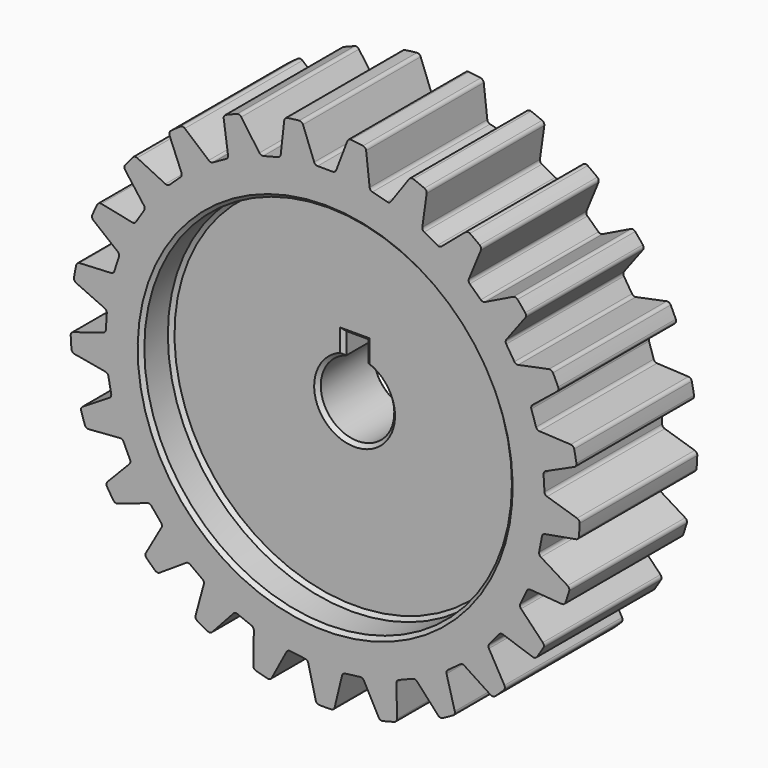
from build123d import *

# Parameters (mm, degrees)
F0_W            = 5.08
F0_H            = 20.32
F3_DEPTH        = 12.7
F3_COPIES_COUNT = 25
F4_R            = 0.508
F6_W            = 3.0840537511
F6_H            = 4.5336009935
F7_DEPTH        = 12.7
F8_SIZE         = 0.508


# Not quite as in the source:
# - a feature of the source that left no trace in its solid (it failed there, or was rolled back) is left out
# - a pattern or mirror of a feature is missing from the dataset's text; its kind, count and spacing are read off the source's solid


with BuildPart() as f1:
    # F0 (on Right) → F1 (revolve)
    with BuildSketch(Plane.YZ):
        Polygon((0, 35.1908973694), (0, 25.4), (5.08, 25.4), (10.16, 25.4), (10.16, 35.1908973694), align=None)
        with Locations((-2.54, 15.24)):
            Rectangle(F0_W, F0_H)
        with Locations((2.54, 15.24)):
            Rectangle(F0_W, F0_H)
        Polygon((-5.08, 25.4), (0, 25.4), (0, 35.1908973694), (-10.16, 35.1908973694), (-10.16, 25.4), align=None)
    revolve(axis=Axis((0, 8.2993172109, 0), (0, 1, 0)))

    # F2 (on Front) → F3 (cut, symmetric)
    with BuildSketch(Plane.XZ):
        Polygon((3.3019999777, 35.3079517332), (-2.23e-08, 35.3079517332), (-3.3020000223, 35.3079517332), (-1.3963384554, 30.2987862378), (-2.23e-08, 30.2987862378), (1.3963384108, 30.2987862378), align=None)
    f3 = extrude(amount=F3_DEPTH, both=True, mode=Mode.SUBTRACT)

    # F3_copies: F3 ×25 about axis
    f3_copies_axis = Axis((0, 0, 0), (0, 1, 0))
    for i in range(1, F3_COPIES_COUNT):
        add(f3.rotate(f3_copies_axis, i * 360 / F3_COPIES_COUNT), mode=Mode.SUBTRACT)

    # F4
    f4_edges = [f1.edges().sort_by_distance(p)[0] for p in [
        (-1.396338, 0, 30.298786),
        (1.396338, 0, 30.298786),
        (3.201936, 0, 35.044926),
        (-3.201936, 0, 35.044926),
        (-5.613978, 0, 34.740215),
        (-6.182532, 0, 29.694149),
        (-8.887472, 0, 28.999639),
        (-11.81666, 0, 33.147636),
        (-14.077144, 0, 32.252647),
        (-13.372931, 0, 27.22372),
        (-15.820172, 0, 25.878338),
        (-19.6889, 0, 29.167559),
        (-21.655792, 0, 27.738528),
        (-19.72306, 0, 23.042724),
        (-21.758833, 0, 21.131005),
        (-26.324014, 0, 23.354776),
        (-27.873727, 0, 21.481495),
        (-24.833916, 0, 17.413869),
        (-26.330307, 0, 15.055934),
        (-31.305093, 0, 16.074527),
        (-32.340253, 0, 13.8747),
        (-28.384366, 0, 10.690837),
        (-29.24735, 0, 8.034843),
        (-34.319158, 0, 7.784256),
        (-34.774722, 0, 5.396107),
        (-30.151322, 0, 3.29606),
        (-30.326675, 0, 0.508893),
        (-35.176824, 0, -0.995129),
        (-35.024167, 0, -3.421544),
        (-30.023759, 0, -4.305821),
        (-29.500464, 0, -7.049032),
        (-33.824201, 0, -9.711985),
        (-33.072915, 0, -12.024206),
        (-28.009693, 0, -11.637151),
        (-26.820629, 0, -14.164041),
        (-30.346279, 0, -17.818602),
        (-29.043571, 0, -19.871343),
        (-24.235676, 0, -18.237276),
        (-22.455556, 0, -20.38907),
        (-24.961589, 0, -24.805611),
        (-23.189311, 0, -26.46989),
        (-18.938841, 0, -23.691486),
        (-16.679518, 0, -25.33298),
        (-18.00847, 0, -30.233992),
        (-15.877983, 0, -31.405237),
        (-12.45201, 0, -27.657073),
        (-9.855444, 0, -28.685125),
        (-9.923813, 0, -33.76266),
        (-7.568982, 0, -34.367278),
        (-5.182773, 0, -29.884864),
        (-2.412117, 0, -30.234879),
        (-1.215606, 0, -35.169896),
        (1.215606, 0, -35.169896),
        (2.412117, 0, -30.234879),
        (5.182773, 0, -29.884864),
        (7.568982, 0, -34.367278),
        (9.923813, 0, -33.76266),
        (9.855445, 0, -28.685125),
        (12.45201, 0, -27.657073),
        (15.877983, 0, -31.405237),
        (18.00847, 0, -30.233992),
        (16.679518, 0, -25.33298),
        (18.938841, 0, -23.691486),
        (23.189312, 0, -26.46989),
        (24.961589, 0, -24.805611),
        (22.455556, 0, -20.38907),
        (24.235676, 0, -18.237276),
        (29.043571, 0, -19.871343),
        (30.346279, 0, -17.818602),
        (26.820629, 0, -14.164041),
        (28.009693, 0, -11.637151),
        (33.072915, 0, -12.024206),
        (33.824201, 0, -9.711985),
        (29.500464, 0, -7.049032),
        (30.023759, 0, -4.305821),
        (35.024167, 0, -3.421543),
        (35.176824, 0, -0.995129),
        (30.326675, 0, 0.508893),
        (30.151322, 0, 3.29606),
        (34.774722, 0, 5.396107),
        (34.319158, 0, 7.784256),
        (29.24735, 0, 8.034843),
        (28.384366, 0, 10.690837),
        (32.340253, 0, 13.8747),
        (31.305093, 0, 16.074527),
        (26.330307, 0, 15.055934),
        (24.833916, 0, 17.413869),
        (27.873727, 0, 21.481495),
        (26.324014, 0, 23.354776),
        (21.758833, 0, 21.131005),
        (19.72306, 0, 23.042724),
        (21.655792, 0, 27.738528),
        (19.6889, 0, 29.167559),
        (15.820172, 0, 25.878338),
        (13.372931, 0, 27.22372),
        (14.077144, 0, 32.252647),
        (11.81666, 0, 33.147636),
        (8.887472, 0, 28.999639),
        (6.182532, 0, 29.694149),
        (5.613978, 0, 34.740215),
    ]]
    fillet(f4_edges, radius=F4_R)

    # F6 (on Front) → F7 (cut, symmetric)
    with BuildSketch(Plane.XZ):
        with Locations((0, 5.5242006201)):
            Rectangle(F6_W, F6_H)
    extrude(amount=F7_DEPTH, both=True, mode=Mode.SUBTRACT)

    # F8
    f8_edges = [f1.edges().sort_by_distance(p)[0] for p in [
        (0, -5.08, -25.4),
        (0, -10.16, -25.4),
        (0, 5.08, -25.4),
        (0, 10.16, -25.4),
        (0, -5.08, -5.08),
        (-1.542027, -5.08, 6.315653),
        (0, -5.08, 7.791001),
        (1.542027, -5.08, 6.315653),
        (0, 5.08, -5.08),
        (-1.542027, 5.08, 6.315653),
        (0, 5.08, 7.791001),
        (1.542027, 5.08, 6.315653),
    ]]
    chamfer(f8_edges, length=F8_SIZE)


solid = f1.part
